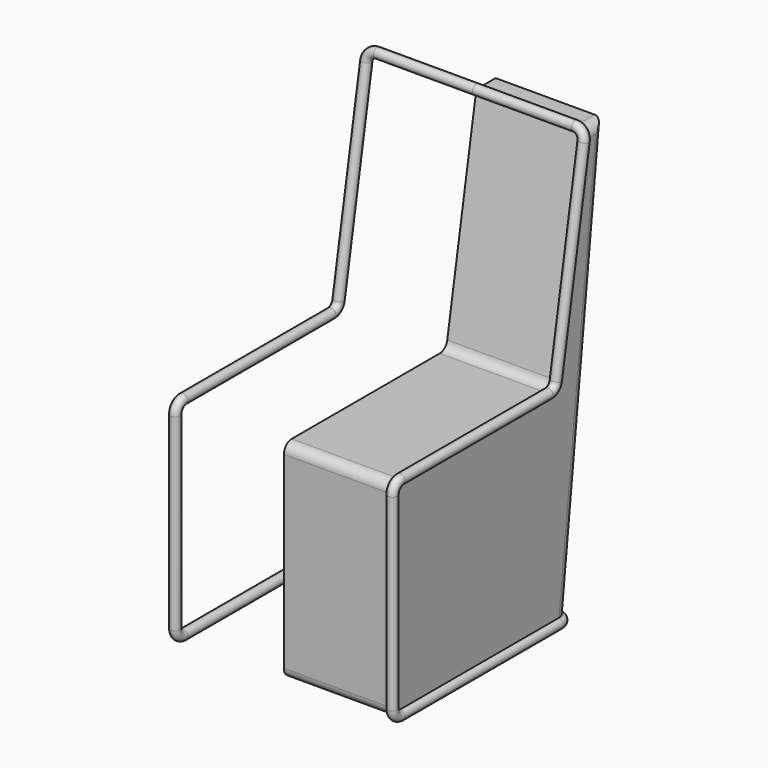
from build123d import *

# Parameters (mm, degrees)
F1_DEPTH = 225
F2_R     = 20
F6_R     = 10


with BuildPart() as f1:
    # F0 (on Right) → F1 (new body)
    with BuildSketch(Plane.YZ):
        Polygon((-450, 0), (0, 0), (98.1416799501, 873.1634888555), (48.1416799501, 873.1634888555), (-30, 430), (-450, 430), align=None)
    extrude(amount=F1_DEPTH)

    # F2
    f2_edges = [f1.edges().sort_by_distance(p)[0] for p in [
        (225, 73.14168, 873.163489),
        (225, 49.07084, 436.581744),
        (112.5, -30, 430),
        (112.5, -450, 430),
        (112.5, -450, 0),
    ]]
    fillet(f2_edges, radius=F2_R)


with BuildPart() as f7:
    # F7: sweep along a path in F5, F3, F4
    with BuildLine(Plane(origin=(0, 0, 0), x_dir=(1, 0, 0), z_dir=(0, 0, -1))) as f7_path:
        Line((0, 0), (205, 0))
        add(Plane(origin=(0, 0, 0), x_dir=(1, 0, 0), z_dir=(0, 0, -1)) * Edge.make_bspline(
            [(205, 0), (225, 0), (225, 20.1259362199)],
            knots=[3.1415926536, 3.1415926536, 3.1415926536, 4.7123889804, 4.7123889804, 4.7123889804], degree=2, weights=[1, 0.7071067812, 1]))
    with BuildLine(Plane.YZ.offset(225)) as f7_path_2:
        Line((-20.1259362199, 0), (-430, 0))
        ThreePointArc((-430, 0), (-444.1421356237, 5.8578643763), (-450, 20))
        Line((-450, 20), (-450, 410))
        ThreePointArc((-450, 410), (-444.1421356237, 424.1421356237), (-430, 430))
        Line((-430, 430), (-46.7819926235, 430))
        ThreePointArc((-46.7819926235, 430), (-33.9262404298, 434.6791111376), (-27.0858375633, 446.5270364467))
        Line((-27.0858375633, 446.5270364467), (44.6151403359, 853.1634888555))
    with BuildLine(Plane(origin=(0, -102.6297201268, 18.0963886809), x_dir=(1, 0, 0), z_dir=(0, -0.984807753, 0.1736481777))) as f7_path_3:
        add(Plane(origin=(0, -102.6297201268, 18.0963886809), x_dir=(1, 0, 0), z_dir=(0, -0.984807753, 0.1736481777)) * Edge.make_bspline(
            [(225, 847.9493562275), (225, 868.2578884652), (205, 868.2578884652)],
            knots=[4.7123889804, 4.7123889804, 4.7123889804, 6.2831853072, 6.2831853072, 6.2831853072], degree=2, weights=[1, 0.7071067812, 1]))
        Line((205, 868.2578884652), (0, 868.2578884652))
    # F6 (on Right) → F7 (sweep)
    with BuildSketch(Plane.YZ):
        Circle(F6_R)
    sweep(path=f7_path.line + f7_path_2.line + f7_path_3.line)

    # F8: F7 across face


with BuildPart() as f7_1:
    add(f7.part)
    add(f7.part.mirror(Plane(origin=(0, 0, 0), x_dir=(0, -1, 0), z_dir=(-1, 0, 0))))


solid = Compound([f1.part, f7_1.part])
